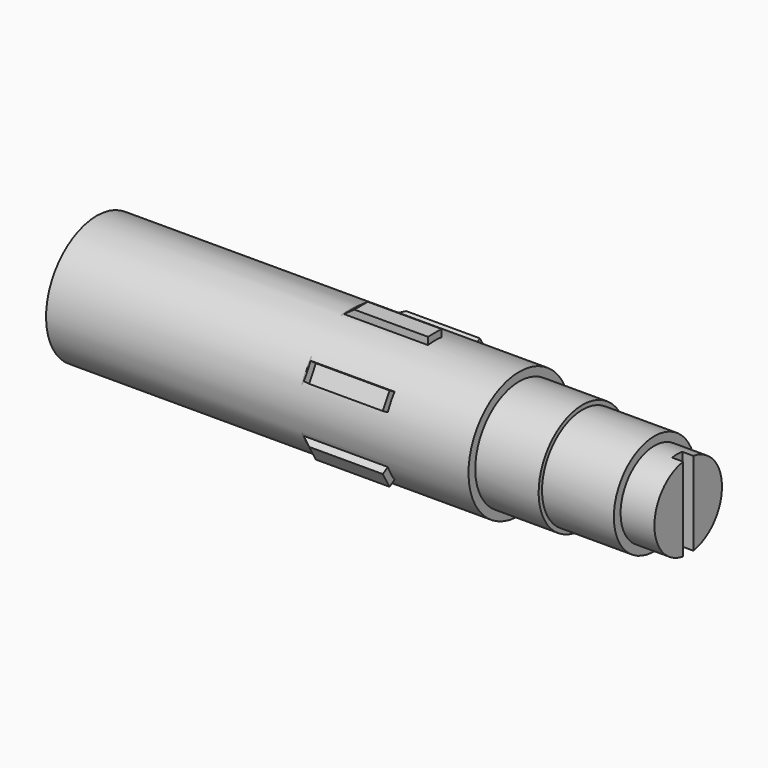
from build123d import *

# Parameters (mm, degrees)
F3_DEPTH        = 1.3
F5_START        = -10
F5_DEPTH        = 10
F5_COPIES_COUNT = 6
F6_T4_DEPTH     = 8.638880276
F6_S5_R         = 7.5
F6_T6_DEPTH     = 6
F6_T10_DEPTH    = 8.638880276
F6_S11_R        = 7.5
F6_T12_DEPTH    = 6
F6_T16_DEPTH    = 8.638880276
F6_S17_R        = 7.5
F6_T18_DEPTH    = 6
F6_T22_DEPTH    = 8.638880276
F6_S23_R        = 7.5
F6_T24_DEPTH    = 6
F6_T28_DEPTH    = 8.638880276
F6_S29_R        = 7.5
F6_T30_DEPTH    = 6
F6_T34_DEPTH    = 8.638880276
F6_S35_R        = 7.5
F6_T36_DEPTH    = 6


# Not quite as in the source:
# - a fillet or chamfer that OpenCascade refuses, or shapes differently, is made with other operations: its cross-section is extruded or revolved along the edge and cut away or added
# - a pattern or mirror of a feature is missing from the dataset's text; its kind, count and spacing are read off the source's solid
# - a feature names something its author has since deleted; it is built from what else it names


with BuildPart() as f1:
    # F0 (on Front) → F1 (revolve)
    with BuildSketch(Plane.XZ):
        Polygon((70, 5), (66, 5), (66, 6), (57.5, 6), (57.5, 6.5), (50, 6.5), (50, 7.5), (0, 7.5), (0, 0), (70, 0), align=None)
    revolve(axis=Axis((22.5240401924, 0, 0), (1, 0, 0)))

    # F2 (on face) → F3 (cut)
    with BuildSketch(Plane.YZ.offset(70)):
        with BuildLine():
            ThreePointArc((0.75, 4.9434299833), (0, 5), (-0.75, 4.9434299833))
            Line((-0.75, 4.9434299833), (-0.75, -4.9434299833))
            ThreePointArc((-0.75, -4.9434299833), (0, -5), (0.75, -4.9434299833))
            Line((0.75, -4.9434299833), (0.75, 4.9434299833))
        make_face()
    extrude(amount=-F3_DEPTH, mode=Mode.SUBTRACT)

    # F4 (on face) → F5 (join)
    with BuildSketch(Plane.YZ.offset(50).offset(F5_START)):
        with BuildLine():
            ThreePointArc((-1, 7.4330343737), (0, 7.5), (1, 7.4330343737))
            Line((1, 7.4330343737), (1, 8.3))
            Line((1, 8.3), (-1, 8.3))
            Line((-1, 8.3), (-1, 7.4330343737))
        make_face()
    f5 = extrude(amount=-F5_DEPTH)

    # F5_copies: F5 ×6 about axis
    f5_copies_axis = Axis((0, 0, 0), (1, 0, 0))
    for i in range(1, F5_COPIES_COUNT):
        add(f5.rotate(f5_copies_axis, i * 360 / F5_COPIES_COUNT))

    # F6: chamfer of 0.9 x 1.2853332061 on 6 edges, made by hand


with BuildPart() as f6_tool2:
    # F6_s3 → F6_t4 (new body)
    with BuildSketch(Plane.XZ.offset(-4.319440138)):
        with BuildLine():
            Line((29.9578846671, 7.3705105264), (31.327448539, 8.3294894736))
            Line((31.327448539, 8.3294894736), (31.327448539, 8.3551961377))
            ThreePointArc((31.327448539, 8.3551961377), (30.6637242695, 8.3257066641), (30, 8.3257066641))
            Line((30, 8.3257066641), (29.9742933359, 8.3))
            ThreePointArc((29.9742933359, 8.3), (29.9742933359, 7.8352552632), (29.9321780029, 7.3705105264))
            Line((29.9321780029, 7.3705105264), (29.9578846671, 7.3705105264))
        make_face()
    extrude(amount=F6_T4_DEPTH)

    # F6_s5 → F6_t6 (cut, symmetric)
    with BuildSketch(Plane.YZ.offset(30.6)):
        Circle(F6_S5_R)
    extrude(amount=F6_T6_DEPTH, both=True, mode=Mode.SUBTRACT)


with BuildPart() as f1_1:
    add(f1.part)

    # F6_t1: cut F6_tool2
    add(f6_tool2.part, mode=Mode.SUBTRACT)


with BuildPart() as f6_tool8:
    # F6_s9 → F6_t10 (new body)
    with BuildSketch(Plane.XZ.offset(4.319440138)):
        with BuildLine():
            Line((31.327448539, -8.3294894736), (29.9578846671, -7.3705105264))
            Line((29.9578846671, -7.3705105264), (29.9321780029, -7.3705105264))
            ThreePointArc((29.9321780029, -7.3705105264), (29.9742933359, -7.8352552632), (29.9742933359, -8.3))
            Line((29.9742933359, -8.3), (30, -8.3257066641))
            ThreePointArc((30, -8.3257066641), (30.6637242695, -8.3257066641), (31.327448539, -8.3551961377))
            Line((31.327448539, -8.3551961377), (31.327448539, -8.3294894736))
        make_face()
    extrude(amount=-F6_T10_DEPTH)

    # F6_s11 → F6_t12 (cut, symmetric)
    with BuildSketch(Plane.YZ.offset(30.6)):
        Circle(F6_S11_R)
    extrude(amount=F6_T12_DEPTH, both=True, mode=Mode.SUBTRACT)


with BuildPart() as f1_2:
    add(f1_1.part)

    # F6_t7: cut F6_tool8
    add(f6_tool8.part, mode=Mode.SUBTRACT)


with BuildPart() as f6_tool14:
    # F6_s15 → F6_t16 (new body)
    with BuildSketch(Plane(origin=(0, -2.159720069, 3.7407448896), x_dir=(1, 0, 0), z_dir=(0, 0.5, -0.8660254038))):
        with BuildLine():
            Line((29.9578846671, 7.3705105264), (31.327448539, 8.3294894736))
            Line((31.327448539, 8.3294894736), (31.327448539, 8.3551961377))
            ThreePointArc((31.327448539, 8.3551961377), (30.6637242695, 8.3257066641), (30, 8.3257066641))
            Line((30, 8.3257066641), (29.9742933359, 8.3))
            ThreePointArc((29.9742933359, 8.3), (29.9742933359, 7.8352552632), (29.9321780029, 7.3705105264))
            Line((29.9321780029, 7.3705105264), (29.9578846671, 7.3705105264))
        make_face()
    extrude(amount=F6_T16_DEPTH)

    # F6_s17 → F6_t18 (cut, symmetric)
    with BuildSketch(Plane.YZ.offset(30.6)):
        Circle(F6_S17_R)
    extrude(amount=F6_T18_DEPTH, both=True, mode=Mode.SUBTRACT)


with BuildPart() as f1_3:
    add(f1_2.part)

    # F6_t13: cut F6_tool14
    add(f6_tool14.part, mode=Mode.SUBTRACT)


with BuildPart() as f6_tool20:
    # F6_s21 → F6_t22 (new body)
    with BuildSketch(Plane(origin=(0, 2.159720069, 3.7407448896), x_dir=(1, 0, 0), z_dir=(0, -0.5, -0.8660254038))):
        with BuildLine():
            Line((29.9578846671, 7.3705105264), (31.327448539, 8.3294894736))
            Line((31.327448539, 8.3294894736), (31.327448539, 8.3551961377))
            ThreePointArc((31.327448539, 8.3551961377), (30.6637242695, 8.3257066641), (30, 8.3257066641))
            Line((30, 8.3257066641), (29.9742933359, 8.3))
            ThreePointArc((29.9742933359, 8.3), (29.9742933359, 7.8352552632), (29.9321780029, 7.3705105264))
            Line((29.9321780029, 7.3705105264), (29.9578846671, 7.3705105264))
        make_face()
    extrude(amount=F6_T22_DEPTH)

    # F6_s23 → F6_t24 (cut, symmetric)
    with BuildSketch(Plane.YZ.offset(30.6)):
        Circle(F6_S23_R)
    extrude(amount=F6_T24_DEPTH, both=True, mode=Mode.SUBTRACT)


with BuildPart() as f1_4:
    add(f1_3.part)

    # F6_t19: cut F6_tool20
    add(f6_tool20.part, mode=Mode.SUBTRACT)


with BuildPart() as f6_tool26:
    # F6_s27 → F6_t28 (new body)
    with BuildSketch(Plane(origin=(0, -2.159720069, -3.7407448896), x_dir=(1, 0, 0), z_dir=(0, 0.5, 0.8660254038))):
        with BuildLine():
            Line((29.9578846671, 7.3705105264), (31.327448539, 8.3294894736))
            Line((31.327448539, 8.3294894736), (31.327448539, 8.3551961377))
            ThreePointArc((31.327448539, 8.3551961377), (30.6637242695, 8.3257066641), (30, 8.3257066641))
            Line((30, 8.3257066641), (29.9742933359, 8.3))
            ThreePointArc((29.9742933359, 8.3), (29.9742933359, 7.8352552632), (29.9321780029, 7.3705105264))
            Line((29.9321780029, 7.3705105264), (29.9578846671, 7.3705105264))
        make_face()
    extrude(amount=F6_T28_DEPTH)

    # F6_s29 → F6_t30 (cut, symmetric)
    with BuildSketch(Plane.YZ.offset(30.6)):
        Circle(F6_S29_R)
    extrude(amount=F6_T30_DEPTH, both=True, mode=Mode.SUBTRACT)


with BuildPart() as f1_5:
    add(f1_4.part)

    # F6_t25: cut F6_tool26
    add(f6_tool26.part, mode=Mode.SUBTRACT)


with BuildPart() as f6_tool32:
    # F6_s33 → F6_t34 (new body)
    with BuildSketch(Plane(origin=(0, 2.159720069, -3.7407448896), x_dir=(1, 0, 0), z_dir=(0, -0.5, 0.8660254038))):
        with BuildLine():
            Line((29.9578846671, 7.3705105264), (31.327448539, 8.3294894736))
            Line((31.327448539, 8.3294894736), (31.327448539, 8.3551961377))
            ThreePointArc((31.327448539, 8.3551961377), (30.6637242695, 8.3257066641), (30, 8.3257066641))
            Line((30, 8.3257066641), (29.9742933359, 8.3))
            ThreePointArc((29.9742933359, 8.3), (29.9742933359, 7.8352552632), (29.9321780029, 7.3705105264))
            Line((29.9321780029, 7.3705105264), (29.9578846671, 7.3705105264))
        make_face()
    extrude(amount=F6_T34_DEPTH)

    # F6_s35 → F6_t36 (cut, symmetric)
    with BuildSketch(Plane.YZ.offset(30.6)):
        Circle(F6_S35_R)
    extrude(amount=F6_T36_DEPTH, both=True, mode=Mode.SUBTRACT)


with BuildPart() as f1_6:
    add(f1_5.part)

    # F6_t31: cut F6_tool32
    add(f6_tool32.part, mode=Mode.SUBTRACT)


solid = f1_6.part
